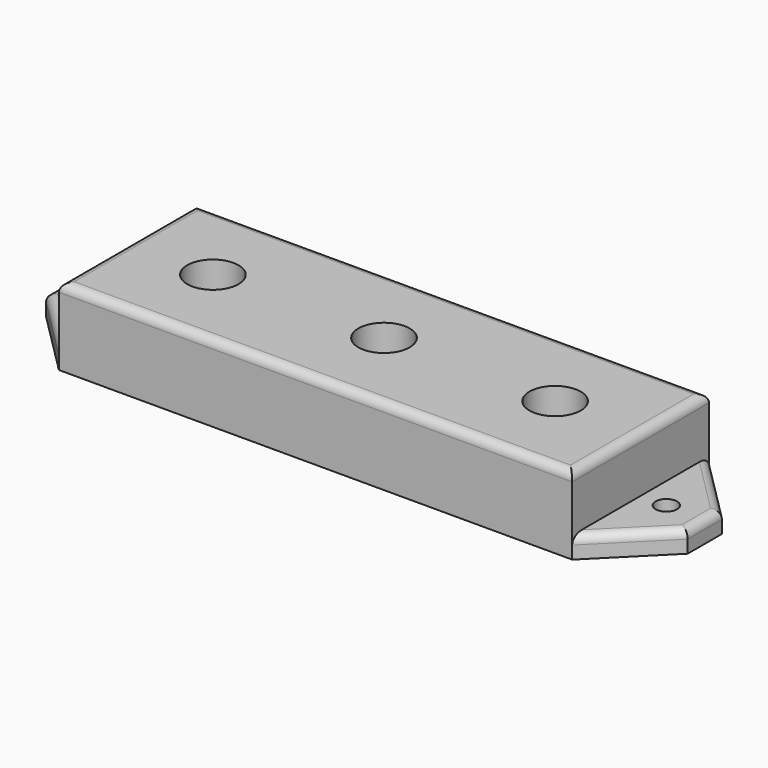
from build123d import *

# Parameters (mm, degrees)
F0_W        = 76.2
F0_H        = 25.4
F1_DEPTH    = 11.43
F2_R        = 3.81
F3_DEPTH    = 6.35
F4_R        = 1.27
F5_W        = 25.4
F5_H        = 3.175
F6_DEPTH    = 9.525
F7_W        = 25.4
F7_H        = 3.175
F8_DEPTH    = 9.525
F9_T1_DEPTH = 52.1655609208
F10_R       = 1.27
F11_R       = 1.5875
F12_DEPTH   = 25.4
F13_R       = 1.5875
F14_DEPTH   = 25.4


# Not quite as in the source:
# - a fillet or chamfer that OpenCascade refuses, or shapes differently, is made with other operations: its cross-section is extruded or revolved along the edge and cut away or added


with BuildPart() as f1:
    # F0 (on Top) → F1 (new body)
    with BuildSketch(Plane.XY):
        with Locations((38.1, 12.7)):
            Rectangle(F0_W, F0_H)
    extrude(amount=F1_DEPTH)

    # F2 (on face) → F3 (cut)
    with BuildSketch(Plane.XY.offset(11.43)):
        with Locations((12.7, 12.7)):
            Circle(F2_R)
        with Locations((38.1, 12.7)):
            Circle(F2_R)
        with Locations((63.5, 12.7)):
            Circle(F2_R)
    extrude(amount=-F3_DEPTH, mode=Mode.SUBTRACT)

    # F4
    f4_edges = [f1.edges().sort_by_distance(p)[0] for p in [
        (38.1, 0, 11.43),
        (76.2, 12.7, 11.43),
        (38.1, 25.4, 11.43),
        (0, 12.7, 11.43),
    ]]
    fillet(f4_edges, radius=F4_R)

    # F5 (on face) → F6 (join)
    with BuildSketch(Plane.YZ.offset(76.2)):
        with Locations((12.7, 1.5875)):
            Rectangle(F5_W, F5_H)
    extrude(amount=F6_DEPTH)

    # F7 (on face) → F8 (join)
    with BuildSketch(Plane(origin=(0, 0, 0), x_dir=(0, -1, 0), z_dir=(-1, 0, 0))):
        with Locations((-12.7, 1.5875)):
            Rectangle(F7_W, F7_H)
    extrude(amount=F8_DEPTH)

    # F9: chamfer of 9.525 on 6 edges, made by hand

    # F9_s2 → F9_t1 (cut)
    with BuildSketch(Plane.XY.offset(-24.4952804604)):
        Polygon((0, 25.4), (-9.525, 15.875), (-9.525, 25.4), align=None)
        Polygon((76.2, 25.4), (85.725, 15.875), (85.725, 25.4), align=None)
        Polygon((85.725, 9.525), (76.2, 0), (85.725, 0), align=None)
        Polygon((-9.525, 9.525), (0, 0), (-9.525, 0), align=None)
    extrude(amount=F9_T1_DEPTH, mode=Mode.SUBTRACT)

    # F10
    f10_edges = [f1.edges().sort_by_distance(p)[0] for p in [
        (-4.7625, 4.7625, 3.175),
        (-9.525, 12.7, 3.175),
        (-4.7625, 20.6375, 3.175),
        (80.9625, 4.7625, 3.175),
        (85.725, 12.7, 3.175),
        (80.9625, 20.6375, 3.175),
    ]]
    fillet(f10_edges, radius=F10_R)

    # F11 (on face) → F12 (cut)
    with BuildSketch(Plane.XY.offset(3.175)):
        with Locations((-3.81, 12.7)):
            Circle(F11_R)
    extrude(amount=-F12_DEPTH, mode=Mode.SUBTRACT)

    # F13 (on face) → F14 (cut)
    with BuildSketch(Plane.XY.offset(3.175)):
        with Locations((80.01, 12.7)):
            Circle(F13_R)
    extrude(amount=-F14_DEPTH, mode=Mode.SUBTRACT)


solid = f1.part
